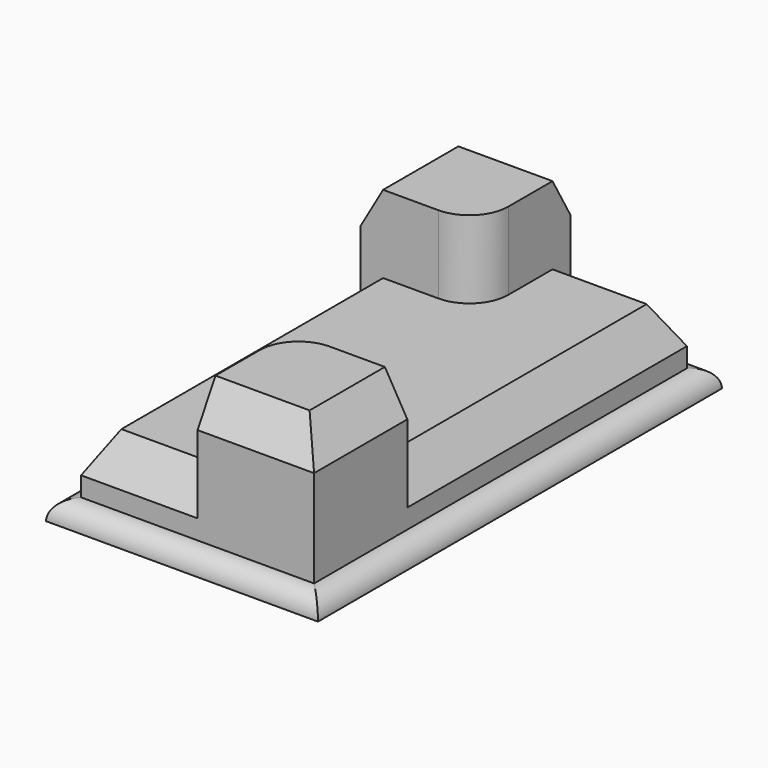
from build123d import *

# Parameters (mm, degrees)
F0_W        = 88.9
F0_H        = 165.1
F1_DEPTH    = 6.35
F2_DEPTH    = 50.8
F3_DEPTH    = 25.4
F4_R        = 6.34999
F5_SIZE2    = 7.3323484187
F5_SIZE     = 12.7
F6_C1_SIZE2 = 7.3323484187
F6_C1_SIZE  = 12.7
F6_C2_SIZE2 = 7.3323484187
F6_C2_SIZE  = 12.7
F6_C3_SIZE2 = 7.3323484187
F6_C3_SIZE  = 12.7


# Not quite as in the source:
# - a fillet or chamfer is up to 0.001 mm smaller than in the source, because OpenCascade refuses the exact size


with BuildPart() as f1:
    # F0 (on Top) → F1 (new body)
    with BuildSketch(Plane.XY):
        Rectangle(F0_W, F0_H)
        Polygon((38.1, -38.1), (38.1, -76.2), (0, -76.2), (-38.1, -76.2), (-38.1, 38.1), (-38.1, 76.2), (0, 76.2), (38.1, 76.2), align=None, mode=Mode.SUBTRACT)
    extrude(amount=F1_DEPTH)

    # F0 (on Top) → F2 (join)
    with BuildSketch(Plane.XY):
        with BuildLine():
            Line((-38.1, 76.2), (-38.1, 38.1))
            Line((-38.1, 38.1), (-12.7, 38.1))
            ThreePointArc((-12.7, 38.1), (-3.7197438789, 41.8197438789), (0, 50.8))
            Line((0, 50.8), (0, 76.2))
            Line((0, 76.2), (-38.1, 76.2))
        make_face()
        with BuildLine():
            Line((0, -76.2), (38.1, -76.2))
            Line((38.1, -76.2), (38.1, -38.1))
            Line((38.1, -38.1), (12.7, -38.1))
            ThreePointArc((12.7, -38.1), (3.7197438789, -41.8197438789), (0, -50.8))
            Line((0, -50.8), (0, -76.2))
        make_face()
    extrude(amount=F2_DEPTH)

    # F0 (on Top) → F3 (join)
    with BuildSketch(Plane.XY):
        with BuildLine():
            Line((-38.1, -76.2), (0, -76.2))
            Line((0, -76.2), (0, -50.8))
            ThreePointArc((0, -50.8), (3.7197438789, -41.8197438789), (12.7, -38.1))
            Line((12.7, -38.1), (38.1, -38.1))
            Line((38.1, -38.1), (38.1, 76.2))
            Line((38.1, 76.2), (0, 76.2))
            Line((0, 76.2), (0, 50.8))
            ThreePointArc((0, 50.8), (-3.7197438789, 41.8197438789), (-12.7, 38.1))
            Line((-12.7, 38.1), (-38.1, 38.1))
            Line((-38.1, 38.1), (-38.1, -76.2))
        make_face()
    extrude(amount=F3_DEPTH)

    # F4 (radius 6.35 in the source; OpenCascade refuses exactly that, so slightly less here)
    f4_edges = [f1.edges().sort_by_distance(p)[0] for p in [
        (0, -82.55, 6.35),
        (-44.45, 0, 6.35),
        (0, 82.55, 6.35),
        (44.45, 0, 6.35),
    ]]
    fillet(f4_edges, radius=F4_R)

    # F5
    f5_edges = [f1.edges().sort_by_distance(p)[0] for p in [
        (-19.05, 76.2, 50.8),
        (-38.1, 57.15, 50.8),
        (38.1, -57.15, 50.8),
        (38.1, 19.05, 25.4),
        (19.05, 76.2, 25.4),
    ]]
    chamfer(f5_edges, length=F5_SIZE, length2=F5_SIZE2)

    # F6: chamfer of 12.7 x 7.3323484187 on 3 edges, made by hand

    # F6_c1
    f6_c1_edges = [f1.edges().sort_by_distance(p)[0] for p in [
        (15.3838257906, -76.2, 50.8),
    ]]
    f6_c1_side = f1.faces().sort_by_distance((15.3838257906, -76.2, 50.6533530316))[0]
    chamfer(f6_c1_edges, length=F6_C1_SIZE, length2=F6_C1_SIZE2, reference=f6_c1_side)

    # F6_c2
    f6_c2_edges = [f1.edges().sort_by_distance(p)[0] for p in [
        (-19.05, -76.2, 25.4),
    ]]
    f6_c2_side = f1.faces().sort_by_distance((-19.05, -76.2, 25.2533530316))[0]
    chamfer(f6_c2_edges, length=F6_C2_SIZE, length2=F6_C2_SIZE2, reference=f6_c2_side)

    # F6_c3
    f6_c3_edges = [f1.edges().sort_by_distance(p)[0] for p in [
        (-38.1, -15.3838257906, 25.4),
    ]]
    f6_c3_side = f1.faces().sort_by_distance((-38.1, -15.3838257906, 25.2533530316))[0]
    chamfer(f6_c3_edges, length=F6_C3_SIZE, length2=F6_C3_SIZE2, reference=f6_c3_side)


solid = f1.part
